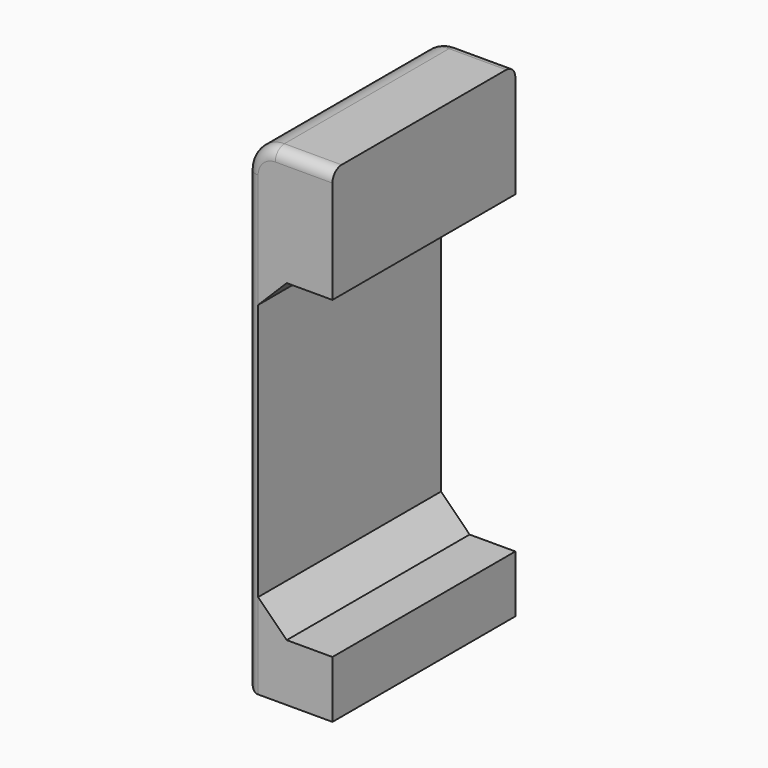
from build123d import *

# Parameters (mm, degrees)
F1_DEPTH = 40
F2_SIZE  = 5
F3_R     = 5
F4_R     = 1.99999


# Not quite as in the source:
# - a fillet or chamfer is up to 0.001 mm smaller than in the source, because OpenCascade refuses the exact size


with BuildPart() as f1:
    # F0 (on Front) → F1 (new body)
    with BuildSketch(Plane.XZ):
        Polygon((-13, 36.2413817516), (-15, 36.2413817516), (-15, -28.7586182484), (0, -28.7586182484), (0, -18.7586182484), (-13, -18.7586182484), align=None)
        Polygon((0, 36.2413817516), (0, 56.2413817516), (-15, 56.2413817516), (-15, 36.2413817516), (-13, 36.2413817516), align=None)
    extrude(amount=F1_DEPTH)

    # F2
    f2_edges = [f1.edges().sort_by_distance(p)[0] for p in [
        (-13, -20, -18.758618),
        (-13, -20, 36.241382),
    ]]
    chamfer(f2_edges, length=F2_SIZE)

    # F3
    f3_edges = [f1.edges().sort_by_distance(p)[0] for p in [
        (-15, -20, 56.241382),
    ]]
    fillet(f3_edges, radius=F3_R)

    # F4 (radius 2 in the source; OpenCascade refuses exactly that, so slightly less here)
    f4_edges = [f1.edges().sort_by_distance(p)[0] for p in [
        (-15, 0, 11.241382),
        (-15, -20, 51.241382),
        (-15, -20, -28.758618),
        (-15, -40, 11.241382),
    ]]
    fillet(f4_edges, radius=F4_R)


solid = f1.part
